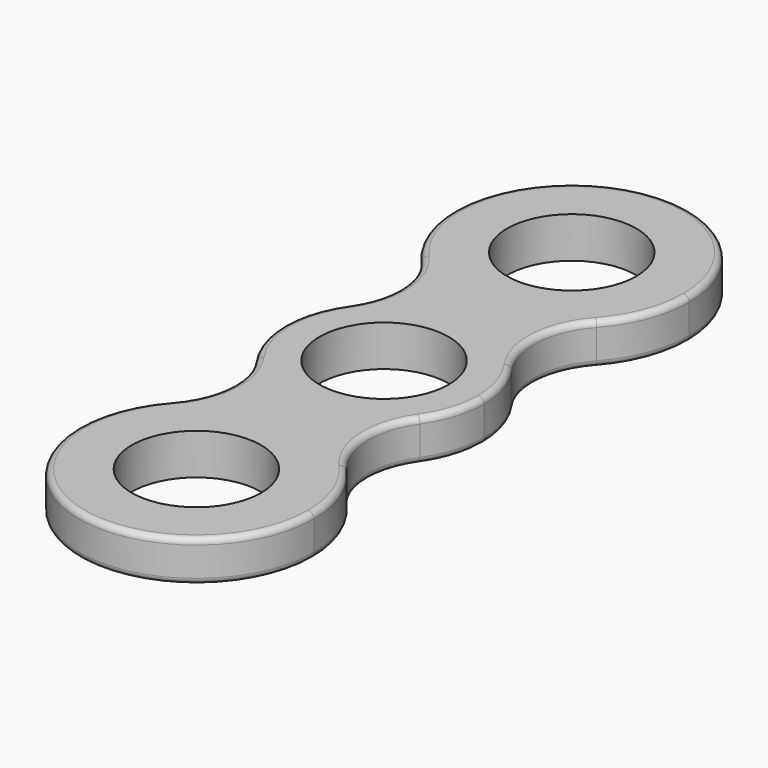
from build123d import *

# Parameters (mm, degrees)
F0_R     = 11.025
F1_DEPTH = 7
F2_R     = 1


# Not quite as in the source:
# - a feature names something its author has since deleted; it is built from what else it names


with BuildPart() as f1:
    # F0 (on Top) → F1 (new body)
    with BuildSketch(Plane.XY):
        with BuildLine():
            ThreePointArc((14.9370437515, 26.6626333571), (18.7098226358, 32.8625521411), (20.025, 40))
            ThreePointArc((20.025, 40), (-7.1374478589, 58.7098226358), (-14.9370437515, 26.6626333571))
            ThreePointArc((-14.9370437515, 26.6626333571), (0, 19.975), (14.9370437515, 26.6626333571))
        make_face()
        with Locations((0, 40)):
            Circle(F0_R, mode=Mode.SUBTRACT)
        with BuildLine():
            ThreePointArc((14.9370437515, 26.6626333571), (0, 19.975), (-14.9370437515, 26.6626333571))
            ThreePointArc((-14.9370437515, 26.6626333571), (-11.4991266725, 18.3897005812), (-13.9423398463, 9.7704546778))
            ThreePointArc((-13.9423398463, 9.7704546778), (0, 17.025), (13.9423398463, 9.7704546778))
            ThreePointArc((13.9423398463, 9.7704546778), (11.4991266725, 18.3897005812), (14.9370437515, 26.6626333571))
        make_face()
        with BuildLine():
            ThreePointArc((13.9423398463, 9.7704546778), (0, 17.025), (-13.9423398463, 9.7704546778))
            ThreePointArc((-13.9423398463, 9.7704546778), (-17.025, 0), (-13.9423398463, -9.7704546778))
            ThreePointArc((-13.9423398463, -9.7704546778), (0, -17.025), (13.9423398463, -9.7704546778))
            ThreePointArc((13.9423398463, -9.7704546778), (16.2360549531, -5.1226111075), (17.025, 0))
            ThreePointArc((17.025, 0), (16.2360549531, 5.1226111075), (13.9423398463, 9.7704546778))
        make_face()
        Circle(F0_R, mode=Mode.SUBTRACT)
        with BuildLine():
            ThreePointArc((13.9423398463, -9.7704546778), (0, -17.025), (-13.9423398463, -9.7704546778))
            ThreePointArc((-13.9423398463, -9.7704546778), (-11.4991266725, -18.3897005812), (-14.9370437515, -26.6626333571))
            ThreePointArc((-14.9370437515, -26.6626333571), (0, -19.975), (14.9370437515, -26.6626333571))
            ThreePointArc((14.9370437515, -26.6626333571), (11.4991266725, -18.3897005812), (13.9423398463, -9.7704546778))
        make_face()
        with BuildLine():
            ThreePointArc((14.9370437515, -26.6626333571), (0, -19.975), (-14.9370437515, -26.6626333571))
            ThreePointArc((-14.9370437515, -26.6626333571), (-7.1374478589, -58.7098226358), (20.025, -40))
            ThreePointArc((20.025, -40), (18.7098226358, -32.8625521411), (14.9370437515, -26.6626333571))
        make_face()
        with Locations((0, -40)):
            Circle(F0_R, mode=Mode.SUBTRACT)
    extrude(amount=F1_DEPTH)

    # F2
    f2_edges = [f1.edges().sort_by_distance(p)[0] for p in [
        (14.937044, 26.662633, 3.5),
        (-14.937044, 26.662633, 3.5),
        (0, 60.025, 0),
        (0, 60.025, 7),
        (-13.94234, 9.770455, 3.5),
        (-11.499127, 18.389701, 0),
        (-11.499127, 18.389701, 7),
        (-13.94234, -9.770455, 3.5),
        (-14.937044, -26.662633, 3.5),
        (-11.499127, -18.389701, 0),
        (-11.499127, -18.389701, 7),
        (14.937044, -26.662633, 3.5),
        (0, -60.025, 0),
        (0, -60.025, 7),
    ]]
    fillet(f2_edges, radius=F2_R)


solid = f1.part
